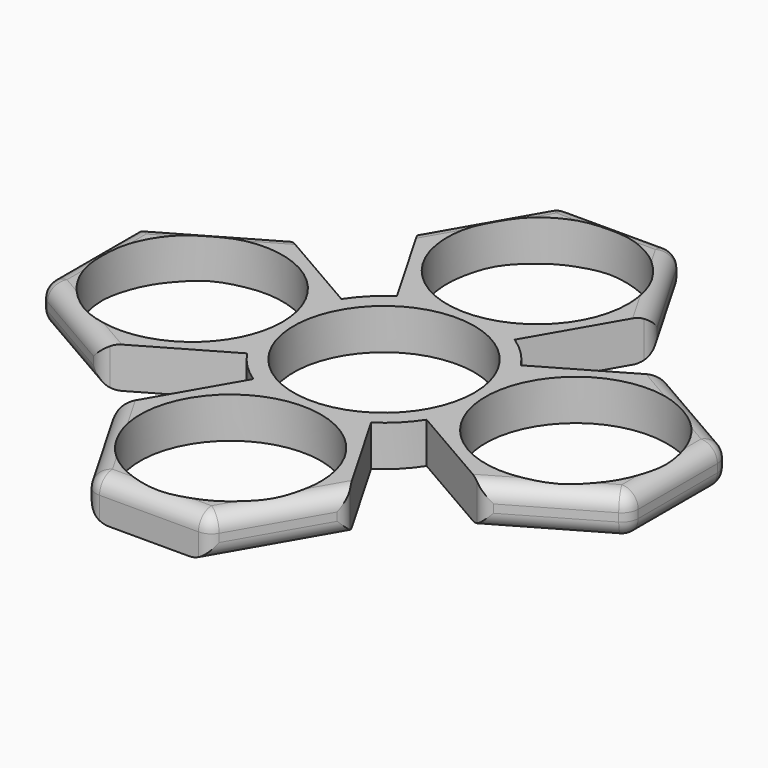
from build123d import *

# Parameters (mm, degrees)
F1_DEPTH      = 5
F2_R          = 11.075
F3_DEPTH      = 5
F4_T1_DEPTH   = 5.8867513459
F4_T3_DEPTH   = 10.7735026919
F4_T5_DEPTH   = 1
F4_T7_DEPTH   = 12.124355653
F4_T9_DEPTH   = 18.2790561914
F4_T11_DEPTH  = 18.2790561914
F4_T13_DEPTH  = 24.4337567297
F4_T15_DEPTH  = 12.124355653
F4_T17_DEPTH  = 24.4337567297
F4_T19_DEPTH  = 18.2790561914
F4_T21_DEPTH  = 18.2790561914
F4_T23_DEPTH  = 18.2790561914
F4_T25_DEPTH  = 24.4337567297
F4_T27_DEPTH  = 18.2790561914
F4_T29_DEPTH  = 18.2790561914
F4_T31_DEPTH  = 18.2790561914
F4_T36_DEPTH  = 2
F4_T42_DEPTH  = 2
F4_T48_DEPTH  = 2
F4_T54_DEPTH  = 2
F4_T60_DEPTH  = 2
F4_T66_DEPTH  = 2
F4_T72_DEPTH  = 2
F4_T78_DEPTH  = 2
F4_T84_DEPTH  = 2
F4_T90_DEPTH  = 2
F4_T96_DEPTH  = 2
F4_T102_DEPTH = 2


# Not quite as in the source:
# - a fillet or chamfer that OpenCascade refuses, or shapes differently, is made with other operations: its cross-section is extruded or revolved along the edge and cut away or added


with BuildPart() as f1:
    # F0 (on Top) → F1 (new body)
    with BuildSketch(Plane.XY):
        with BuildLine():
            ThreePointArc((-11, -7.2057268891), (-13.15, 0), (-11, 7.2057268891))
            Line((-11, 7.2057268891), (-11, 7.2168783649))
            Line((-11, 7.2168783649), (-23.5, 14.4337567297))
            Line((-23.5, 14.4337567297), (-36, 7.2168783649))
            Line((-36, 7.2168783649), (-36, -7.2168783649))
            Line((-36, -7.2168783649), (-23.5, -14.4337567297))
            Line((-23.5, -14.4337567297), (-11, -7.2168783649))
            Line((-11, -7.2168783649), (-11, -7.2057268891))
        make_face()
        with BuildLine():
            ThreePointArc((0, -11), (7.7781745931, -7.7781745931), (11, 0))
            ThreePointArc((11, 0), (7.7781745931, 7.7781745931), (0, 11))
            ThreePointArc((0, 11), (-7.7781745931, 7.7781745931), (-11, 0))
            ThreePointArc((-11, 0), (-7.7781745931, -7.7781745931), (0, -11))
        make_face()
        with BuildLine():
            Line((-11, -7.2057268891), (-11, 0))
            Line((-11, 0), (-11, 7.2057268891))
            ThreePointArc((-11, 7.2057268891), (-13.15, 0), (-11, -7.2057268891))
        make_face()
        with BuildLine():
            ThreePointArc((-7.2057268891, 11), (0, 13.15), (7.2057268891, 11))
            Line((7.2057268891, 11), (7.2168783649, 11))
            Line((7.2168783649, 11), (14.4337567297, 23.5))
            Line((14.4337567297, 23.5), (7.2168783649, 36))
            Line((7.2168783649, 36), (-7.2168783649, 36))
            Line((-7.2168783649, 36), (-14.4337567297, 23.5))
            Line((-14.4337567297, 23.5), (-7.2168783649, 11))
            Line((-7.2168783649, 11), (-7.2057268891, 11))
        make_face()
        with BuildLine():
            ThreePointArc((7.2057268891, -11), (0, -13.15), (-7.2057268891, -11))
            Line((-7.2057268891, -11), (-7.2168783649, -11))
            Line((-7.2168783649, -11), (-14.4337567297, -23.5))
            Line((-14.4337567297, -23.5), (-7.2168783649, -36))
            Line((-7.2168783649, -36), (7.2168783649, -36))
            Line((7.2168783649, -36), (14.4337567297, -23.5))
            Line((14.4337567297, -23.5), (7.2168783649, -11))
            Line((7.2168783649, -11), (7.2057268891, -11))
        make_face()
        with BuildLine():
            ThreePointArc((0, 11), (7.7781745931, 7.7781745931), (11, 0))
            Line((11, 0), (11, 7.2057268891))
            ThreePointArc((11, 7.2057268891), (9.2984541726, 9.2984541726), (7.2057268891, 11))
            Line((7.2057268891, 11), (0, 11))
        make_face()
        with BuildLine():
            ThreePointArc((13.15, 0), (12.6010416236, -3.7598204744), (11, -7.2057268891))
            Line((11, -7.2057268891), (11, -7.2168783649))
            Line((11, -7.2168783649), (23.5, -14.4337567297))
            Line((23.5, -14.4337567297), (36, -7.2168783649))
            Line((36, -7.2168783649), (36, 7.2168783649))
            Line((36, 7.2168783649), (23.5, 14.4337567297))
            Line((23.5, 14.4337567297), (11, 7.2168783649))
            Line((11, 7.2168783649), (11, 7.2057268891))
            ThreePointArc((11, 7.2057268891), (12.6010416236, 3.7598204744), (13.15, 0))
        make_face()
        with BuildLine():
            Line((11, 7.2057268891), (11, 0))
            Line((11, 0), (11, -7.2057268891))
            ThreePointArc((11, -7.2057268891), (12.6010416236, -3.7598204744), (13.15, 0))
            ThreePointArc((13.15, 0), (12.6010416236, 3.7598204744), (11, 7.2057268891))
        make_face()
        with BuildLine():
            Line((7.2057268891, -11), (0, -11))
            Line((0, -11), (-7.2057268891, -11))
            ThreePointArc((-7.2057268891, -11), (0, -13.15), (7.2057268891, -11))
        make_face()
        with BuildLine():
            Line((-7.2057268891, -11), (0, -11))
            ThreePointArc((0, -11), (-7.7781745931, -7.7781745931), (-11, 0))
            Line((-11, 0), (-11, -7.2057268891))
            ThreePointArc((-11, -7.2057268891), (-9.2984541726, -9.2984541726), (-7.2057268891, -11))
        make_face()
        with BuildLine():
            ThreePointArc((-11, 0), (-7.7781745931, 7.7781745931), (0, 11))
            Line((0, 11), (-7.2057268891, 11))
            ThreePointArc((-7.2057268891, 11), (-9.2984541726, 9.2984541726), (-11, 7.2057268891))
            Line((-11, 7.2057268891), (-11, 0))
        make_face()
        with BuildLine():
            Line((11, -7.2057268891), (11, 0))
            ThreePointArc((11, 0), (7.7781745931, -7.7781745931), (0, -11))
            Line((0, -11), (7.2057268891, -11))
            ThreePointArc((7.2057268891, -11), (9.2984541726, -9.2984541726), (11, -7.2057268891))
        make_face()
        with BuildLine():
            Line((-7.2057268891, 11), (0, 11))
            Line((0, 11), (7.2057268891, 11))
            ThreePointArc((7.2057268891, 11), (0, 13.15), (-7.2057268891, 11))
        make_face()
    extrude(amount=F1_DEPTH)

    # F2 (on face) → F3 (cut)
    with BuildSketch(Plane.XY.offset(5)):
        Circle(F2_R)
        with Locations((0, 23.5)):
            Circle(F2_R)
        with Locations((23.5, 0)):
            Circle(F2_R)
        with Locations((-23.5, 0)):
            Circle(F2_R)
        with Locations((0, -23.5)):
            Circle(F2_R)
    extrude(amount=-F3_DEPTH, mode=Mode.SUBTRACT)

    # F4: fillet of radius 2 on 38 edges, made by hand

    # F4_s2 → F4_t1 (cut)
    with BuildSketch(Plane.XY.offset(-2.8867513459)):
        with BuildLine():
            ThreePointArc((-7.7942286341, -35), (-7.0621778265, -35.7320508076), (-6.0621778265, -36))
            Line((-6.0621778265, -36), (-7.2168783649, -36))
            Line((-7.2168783649, -36), (-7.7942286341, -35))
        make_face()
        with BuildLine():
            ThreePointArc((6.0621778265, -36), (7.0621778265, -35.7320508076), (7.7942286341, -35))
            Line((7.7942286341, -35), (7.2168783649, -36))
            Line((7.2168783649, -36), (6.0621778265, -36))
        make_face()
    extrude(amount=F4_T1_DEPTH, mode=Mode.SUBTRACT)

    # F4_s4 → F4_t3 (cut)
    with BuildSketch(Plane.XY.offset(-2.8867513459)):
        with BuildLine():
            ThreePointArc((13.8564064606, -24.5), (14.124355653, -23.5), (13.8564064606, -22.5))
            Line((13.8564064606, -22.5), (14.4337567297, -23.5))
            Line((14.4337567297, -23.5), (13.8564064606, -24.5))
        make_face()
        with BuildLine():
            ThreePointArc((-13.8564064606, -22.5), (-14.124355653, -23.5), (-13.8564064606, -24.5))
            Line((-13.8564064606, -24.5), (-14.4337567297, -23.5))
            Line((-14.4337567297, -23.5), (-13.8564064606, -22.5))
        make_face()
        with BuildLine():
            ThreePointArc((-24.5, -13.8564064606), (-23.5, -14.124355653), (-22.5, -13.8564064606))
            Line((-22.5, -13.8564064606), (-23.5, -14.4337567297))
            Line((-23.5, -14.4337567297), (-24.5, -13.8564064606))
        make_face()
        with BuildLine():
            ThreePointArc((24.5, -13.8564064606), (23.5, -14.124355653), (22.5, -13.8564064606))
            Line((22.5, -13.8564064606), (23.5, -14.4337567297))
            Line((23.5, -14.4337567297), (24.5, -13.8564064606))
        make_face()
        with BuildLine():
            ThreePointArc((-13.8564064606, 22.5), (-14.124355653, 23.5), (-13.8564064606, 24.5))
            Line((-13.8564064606, 24.5), (-14.4337567297, 23.5))
            Line((-14.4337567297, 23.5), (-13.8564064606, 22.5))
        make_face()
        with BuildLine():
            ThreePointArc((13.8564064606, 24.5), (14.124355653, 23.5), (13.8564064606, 22.5))
            Line((13.8564064606, 22.5), (14.4337567297, 23.5))
            Line((14.4337567297, 23.5), (13.8564064606, 24.5))
        make_face()
        with BuildLine():
            ThreePointArc((-22.5, 13.8564064606), (-23.5, 14.124355653), (-24.5, 13.8564064606))
            Line((-24.5, 13.8564064606), (-23.5, 14.4337567297))
            Line((-23.5, 14.4337567297), (-22.5, 13.8564064606))
        make_face()
        with BuildLine():
            ThreePointArc((22.5, 13.8564064606), (23.5, 14.124355653), (24.5, 13.8564064606))
            Line((24.5, 13.8564064606), (23.5, 14.4337567297))
            Line((23.5, 14.4337567297), (22.5, 13.8564064606))
        make_face()
    extrude(amount=F4_T3_DEPTH, mode=Mode.SUBTRACT)

    # F4_s6 → F4_t5 (cut)
    with BuildSketch(Plane.XY.offset(2)):
        with BuildLine():
            ThreePointArc((-36, -6.0621778265), (-35.7320508076, -7.0621778265), (-35, -7.7942286341))
            Line((-35, -7.7942286341), (-36, -7.2168783649))
            Line((-36, -7.2168783649), (-36, -6.0621778265))
        make_face()
        with BuildLine():
            ThreePointArc((36, -6.0621778265), (35.7320508076, -7.0621778265), (35, -7.7942286341))
            Line((35, -7.7942286341), (36, -7.2168783649))
            Line((36, -7.2168783649), (36, -6.0621778265))
        make_face()
        with BuildLine():
            ThreePointArc((35, 7.7942286341), (35.7320508076, 7.0621778265), (36, 6.0621778265))
            Line((36, 6.0621778265), (36, 7.2168783649))
            Line((36, 7.2168783649), (35, 7.7942286341))
        make_face()
        with BuildLine():
            ThreePointArc((-7.7942286341, 35), (-7.0621778265, 35.7320508076), (-6.0621778265, 36))
            Line((-6.0621778265, 36), (-7.2168783649, 36))
            Line((-7.2168783649, 36), (-7.7942286341, 35))
        make_face()
        with BuildLine():
            ThreePointArc((6.0621778265, 36), (7.0621778265, 35.7320508076), (7.7942286341, 35))
            Line((7.7942286341, 35), (7.2168783649, 36))
            Line((7.2168783649, 36), (6.0621778265, 36))
        make_face()
    extrude(amount=F4_T5_DEPTH, mode=Mode.SUBTRACT)

    # F4_s8 → F4_t7 (cut)
    with BuildSketch(Plane.XZ.offset(-6.0621778265)):
        with BuildLine():
            ThreePointArc((34, 5), (35.4142135624, 4.4142135624), (36, 3))
            Line((36, 3), (36, 5))
            Line((36, 5), (34, 5))
        make_face()
        with BuildLine():
            ThreePointArc((34, 0), (35.4142135624, 0.5857864376), (36, 2))
            Line((36, 2), (36, 0))
            Line((36, 0), (34, 0))
        make_face()
    extrude(amount=F4_T7_DEPTH, mode=Mode.SUBTRACT)

    # F4_s10 → F4_t9 (cut)
    with BuildSketch(Plane(origin=(7.0448729811, 4.067359312, 0), x_dir=(0, 0, 1), z_dir=(0.8660254038, 0.5, 0))):
        with BuildLine():
            ThreePointArc((5, 22.25), (4.4142135624, 23.6642135624), (3, 24.25))
            Line((3, 24.25), (5, 24.25))
            Line((5, 24.25), (5, 22.25))
        make_face()
        with BuildLine():
            ThreePointArc((0, 22.25), (0.5857864376, 23.6642135624), (2, 24.25))
            Line((2, 24.25), (0, 24.25))
            Line((0, 24.25), (0, 22.25))
        make_face()
    extrude(amount=F4_T9_DEPTH, mode=Mode.SUBTRACT)

    # F4_s12 → F4_t11 (cut)
    with BuildSketch(Plane(origin=(-13.2068874077, -22.875, 0), x_dir=(0, 0, 1), z_dir=(0.5, 0.8660254038, 0))):
        with BuildLine():
            ThreePointArc((5, 22.25), (4.4142135624, 23.6642135624), (3, 24.25))
            Line((3, 24.25), (5, 24.25))
            Line((5, 24.25), (5, 22.25))
        make_face()
    extrude(amount=F4_T11_DEPTH, mode=Mode.SUBTRACT)

    # F4_s14 → F4_t13 (cut)
    with BuildSketch(Plane(origin=(-16.2842376769, -28.2051270189, 0), x_dir=(0, 0, 1), z_dir=(0.5, 0.8660254038, 0))):
        with BuildLine():
            ThreePointArc((0, 22.25), (0.5857864376, 23.6642135624), (2, 24.25))
            Line((2, 24.25), (0, 24.25))
            Line((0, 24.25), (0, 22.25))
        make_face()
    extrude(amount=F4_T13_DEPTH, mode=Mode.SUBTRACT)

    # F4_s16 → F4_t15 (cut)
    with BuildSketch(Plane.YZ.offset(-6.0621778265)):
        with BuildLine():
            ThreePointArc((-34, 5), (-35.4142135624, 4.4142135624), (-36, 3))
            Line((-36, 3), (-36, 5))
            Line((-36, 5), (-34, 5))
        make_face()
        with BuildLine():
            ThreePointArc((34, 0), (35.4142135624, 0.5857864376), (36, 2))
            Line((36, 2), (36, 0))
            Line((36, 0), (34, 0))
        make_face()
        with BuildLine():
            ThreePointArc((34, 5), (35.4142135624, 4.4142135624), (36, 3))
            Line((36, 3), (36, 5))
            Line((36, 5), (34, 5))
        make_face()
    extrude(amount=F4_T15_DEPTH, mode=Mode.SUBTRACT)

    # F4_s18 → F4_t17 (cut)
    with BuildSketch(Plane(origin=(4.067359312, -7.0448729811, 0), x_dir=(0, 0, 1), z_dir=(0.5, -0.8660254038, 0))):
        with BuildLine():
            ThreePointArc((0, 22.25), (0.5857864376, 23.6642135624), (2, 24.25))
            Line((2, 24.25), (0, 24.25))
            Line((0, 24.25), (0, 22.25))
        make_face()
    extrude(amount=F4_T17_DEPTH, mode=Mode.SUBTRACT)

    # F4_s20 → F4_t19 (cut)
    with BuildSketch(Plane(origin=(4.067359312, -7.0448729811, 0), x_dir=(0, 0, 1), z_dir=(0.5, -0.8660254038, 0))):
        with BuildLine():
            ThreePointArc((5, 22.25), (4.4142135624, 23.6642135624), (3, 24.25))
            Line((3, 24.25), (5, 24.25))
            Line((5, 24.25), (5, 22.25))
        make_face()
    extrude(amount=F4_T19_DEPTH, mode=Mode.SUBTRACT)

    # F4_s22 → F4_t21 (cut)
    with BuildSketch(Plane(origin=(-22.875, 13.2068874077, 0), x_dir=(0, 0, 1), z_dir=(0.8660254038, -0.5, 0))):
        with BuildLine():
            ThreePointArc((0, 22.25), (0.5857864376, 23.6642135624), (2, 24.25))
            Line((2, 24.25), (0, 24.25))
            Line((0, 24.25), (0, 22.25))
        make_face()
        with BuildLine():
            ThreePointArc((5, 22.25), (4.4142135624, 23.6642135624), (3, 24.25))
            Line((3, 24.25), (5, 24.25))
            Line((5, 24.25), (5, 22.25))
        make_face()
    extrude(amount=F4_T21_DEPTH, mode=Mode.SUBTRACT)

    # F4_s24 → F4_t23 (cut)
    with BuildSketch(Plane.XZ.offset(-12.2168783649)):
        with BuildLine():
            ThreePointArc((-34, 5), (-35.4142135624, 4.4142135624), (-36, 3))
            Line((-36, 3), (-36, 5))
            Line((-36, 5), (-34, 5))
        make_face()
        with BuildLine():
            ThreePointArc((-34, 0), (-35.4142135624, 0.5857864376), (-36, 2))
            Line((-36, 2), (-36, 0))
            Line((-36, 0), (-34, 0))
        make_face()
    extrude(amount=F4_T23_DEPTH, mode=Mode.SUBTRACT)

    # F4_s26 → F4_t25 (cut)
    with BuildSketch(Plane(origin=(-7.0448729811, -4.067359312, 0), x_dir=(0, 0, 1), z_dir=(-0.8660254038, -0.5, 0))):
        with BuildLine():
            ThreePointArc((2, 24.25), (0.5857864376, 23.6642135624), (0, 22.25))
            Line((0, 22.25), (0, 24.25))
            Line((0, 24.25), (2, 24.25))
        make_face()
        with BuildLine():
            ThreePointArc((3, 24.25), (4.4142135624, 23.6642135624), (5, 22.25))
            Line((5, 22.25), (5, 24.25))
            Line((5, 24.25), (3, 24.25))
        make_face()
    extrude(amount=F4_T25_DEPTH, mode=Mode.SUBTRACT)

    # F4_s28 → F4_t27 (cut)
    with BuildSketch(Plane(origin=(13.2068874077, 22.875, 0), x_dir=(0, 0, 1), z_dir=(-0.5, -0.8660254038, 0))):
        with BuildLine():
            ThreePointArc((0, 22.25), (0.5857864376, 23.6642135624), (2, 24.25))
            Line((2, 24.25), (0, 24.25))
            Line((0, 24.25), (0, 22.25))
        make_face()
        with BuildLine():
            ThreePointArc((5, 22.25), (4.4142135624, 23.6642135624), (3, 24.25))
            Line((3, 24.25), (5, 24.25))
            Line((5, 24.25), (5, 22.25))
        make_face()
    extrude(amount=F4_T27_DEPTH, mode=Mode.SUBTRACT)

    # F4_s30 → F4_t29 (cut)
    with BuildSketch(Plane(origin=(-4.067359312, 7.0448729811, 0), x_dir=(0, 0, 1), z_dir=(-0.5, 0.8660254038, 0))):
        with BuildLine():
            ThreePointArc((5, 22.25), (4.4142135624, 23.6642135624), (3, 24.25))
            Line((3, 24.25), (5, 24.25))
            Line((5, 24.25), (5, 22.25))
        make_face()
        with BuildLine():
            ThreePointArc((0, 22.25), (0.5857864376, 23.6642135624), (2, 24.25))
            Line((2, 24.25), (0, 24.25))
            Line((0, 24.25), (0, 22.25))
        make_face()
    extrude(amount=F4_T29_DEPTH, mode=Mode.SUBTRACT)

    # F4_s32 → F4_t31 (cut)
    with BuildSketch(Plane(origin=(22.875, -13.2068874077, 0), x_dir=(0, 0, 1), z_dir=(-0.8660254038, 0.5, 0))):
        with BuildLine():
            ThreePointArc((0, 22.25), (0.5857864376, 23.6642135624), (2, 24.25))
            Line((2, 24.25), (0, 24.25))
            Line((0, 24.25), (0, 22.25))
        make_face()
        with BuildLine():
            ThreePointArc((5, 22.25), (4.4142135624, 23.6642135624), (3, 24.25))
            Line((3, 24.25), (5, 24.25))
            Line((5, 24.25), (5, 22.25))
        make_face()
    extrude(amount=F4_T31_DEPTH, mode=Mode.SUBTRACT)


with BuildPart() as f4_tool34:
    # F4_s35 → F4_t36 (new body)
    with BuildSketch(Plane.XY.offset(3)):
        Polygon((-6.0621778265, -34), (-6.0621778265, -36), (-7.2168783649, -36), (-7.7942286341, -35), align=None)
    extrude(amount=F4_T36_DEPTH)

    # F4_s37 → F4_t38 (revolve, cut)
    with BuildSketch(Plane(origin=(-6.0621778265, -34, 3), x_dir=(0.5, 0.8660254038, 0), z_dir=(0.8660254038, -0.5, 0))):
        with BuildLine():
            ThreePointArc((0, -2), (2, 0), (0, 2))
            Line((0, 2), (0, -2))
        make_face()
    revolve(axis=Axis((-6.0621778265, -34, 3), (0, 0, 1)), mode=Mode.SUBTRACT)


with BuildPart() as f1_1:
    add(f1.part)

    # F4_t33: cut F4_tool34
    add(f4_tool34.part, mode=Mode.SUBTRACT)


with BuildPart() as f4_tool40:
    # F4_s41 → F4_t42 (new body)
    with BuildSketch(Plane.XY.offset(3)):
        Polygon((6.0621778265, -34), (6.0621778265, -36), (7.2168783649, -36), (7.7942286341, -35), align=None)
    extrude(amount=F4_T42_DEPTH)

    # F4_s43 → F4_t44 (revolve, cut)
    with BuildSketch(Plane(origin=(6.0621778265, -34, 3), x_dir=(-0.5, 0.8660254038, 0), z_dir=(0.8660254038, 0.5, 0))):
        with BuildLine():
            ThreePointArc((0, -2), (2, 0), (0, 2))
            Line((0, 2), (0, -2))
        make_face()
    revolve(axis=Axis((6.0621778265, -34, 3), (0, 0, 1)), mode=Mode.SUBTRACT)


with BuildPart() as f1_2:
    add(f1_1.part)

    # F4_t39: cut F4_tool40
    add(f4_tool40.part, mode=Mode.SUBTRACT)


with BuildPart() as f4_tool46:
    # F4_s47 → F4_t48 (new body)
    with BuildSketch(Plane.XY.offset(2)):
        Polygon((-34, -6.0621778265), (-36, -6.0621778265), (-36, -7.2168783649), (-35, -7.7942286341), align=None)
    extrude(amount=-F4_T48_DEPTH)

    # F4_s49 → F4_t50 (revolve, cut)
    with BuildSketch(Plane(origin=(-34, -6.0621778265, 2), x_dir=(0.8660254038, 0.5, 0), z_dir=(-0.5, 0.8660254038, 0))):
        with BuildLine():
            ThreePointArc((0, -2), (2, 0), (0, 2))
            Line((0, 2), (0, -2))
        make_face()
    revolve(axis=Axis((-34, -6.0621778265, 2), (0, 0, -1)), mode=Mode.SUBTRACT)


with BuildPart() as f1_3:
    add(f1_2.part)

    # F4_t45: cut F4_tool46
    add(f4_tool46.part, mode=Mode.SUBTRACT)


with BuildPart() as f4_tool52:
    # F4_s53 → F4_t54 (new body)
    with BuildSketch(Plane.XY.offset(3)):
        Polygon((-34, -6.0621778265), (-36, -6.0621778265), (-36, -7.2168783649), (-35, -7.7942286341), align=None)
    extrude(amount=F4_T54_DEPTH)

    # F4_s55 → F4_t56 (revolve, cut)
    with BuildSketch(Plane(origin=(-34, -6.0621778265, 3), x_dir=(0.8660254038, 0.5, 0), z_dir=(0.5, -0.8660254038, 0))):
        with BuildLine():
            ThreePointArc((0, -2), (2, 0), (0, 2))
            Line((0, 2), (0, -2))
        make_face()
    revolve(axis=Axis((-34, -6.0621778265, 3), (0, 0, 1)), mode=Mode.SUBTRACT)


with BuildPart() as f1_4:
    add(f1_3.part)

    # F4_t51: cut F4_tool52
    add(f4_tool52.part, mode=Mode.SUBTRACT)


with BuildPart() as f4_tool58:
    # F4_s59 → F4_t60 (new body)
    with BuildSketch(Plane.XY.offset(2)):
        Polygon((34, -6.0621778265), (36, -6.0621778265), (36, -7.2168783649), (35, -7.7942286341), align=None)
    extrude(amount=-F4_T60_DEPTH)

    # F4_s61 → F4_t62 (revolve, cut)
    with BuildSketch(Plane(origin=(34, -6.0621778265, 2), x_dir=(-0.8660254038, 0.5, 0), z_dir=(-0.5, -0.8660254038, 0))):
        with BuildLine():
            ThreePointArc((0, -2), (2, 0), (0, 2))
            Line((0, 2), (0, -2))
        make_face()
    revolve(axis=Axis((34, -6.0621778265, 2), (0, 0, -1)), mode=Mode.SUBTRACT)


with BuildPart() as f1_5:
    add(f1_4.part)

    # F4_t57: cut F4_tool58
    add(f4_tool58.part, mode=Mode.SUBTRACT)


with BuildPart() as f4_tool64:
    # F4_s65 → F4_t66 (new body)
    with BuildSketch(Plane.XY.offset(3)):
        Polygon((34, -6.0621778265), (36, -6.0621778265), (36, -7.2168783649), (35, -7.7942286341), align=None)
    extrude(amount=F4_T66_DEPTH)

    # F4_s67 → F4_t68 (revolve, cut)
    with BuildSketch(Plane(origin=(34, -6.0621778265, 3), x_dir=(-0.8660254038, 0.5, 0), z_dir=(0.5, 0.8660254038, 0))):
        with BuildLine():
            ThreePointArc((0, -2), (2, 0), (0, 2))
            Line((0, 2), (0, -2))
        make_face()
    revolve(axis=Axis((34, -6.0621778265, 3), (0, 0, 1)), mode=Mode.SUBTRACT)


with BuildPart() as f1_6:
    add(f1_5.part)

    # F4_t63: cut F4_tool64
    add(f4_tool64.part, mode=Mode.SUBTRACT)


with BuildPart() as f4_tool70:
    # F4_s71 → F4_t72 (new body)
    with BuildSketch(Plane.XY.offset(2)):
        Polygon((34, 6.0621778265), (35, 7.7942286341), (36, 7.2168783649), (36, 6.0621778265), align=None)
    extrude(amount=-F4_T72_DEPTH)

    # F4_s73 → F4_t74 (revolve, cut)
    with BuildSketch(Plane(origin=(34, 6.0621778265, 2), x_dir=(-0.8660254038, -0.5, 0), z_dir=(0.5, -0.8660254038, 0))):
        with BuildLine():
            ThreePointArc((0, -2), (2, 0), (0, 2))
            Line((0, 2), (0, -2))
        make_face()
    revolve(axis=Axis((34, 6.0621778265, 2), (0, 0, -1)), mode=Mode.SUBTRACT)


with BuildPart() as f1_7:
    add(f1_6.part)

    # F4_t69: cut F4_tool70
    add(f4_tool70.part, mode=Mode.SUBTRACT)


with BuildPart() as f4_tool76:
    # F4_s77 → F4_t78 (new body)
    with BuildSketch(Plane.XY.offset(3)):
        Polygon((34, 6.0621778265), (36, 6.0621778265), (36, 7.2168783649), (35, 7.7942286341), align=None)
    extrude(amount=F4_T78_DEPTH)

    # F4_s79 → F4_t80 (revolve, cut)
    with BuildSketch(Plane(origin=(34, 6.0621778265, 3), x_dir=(-0.8660254038, -0.5, 0), z_dir=(-0.5, 0.8660254038, 0))):
        with BuildLine():
            ThreePointArc((0, -2), (2, 0), (0, 2))
            Line((0, 2), (0, -2))
        make_face()
    revolve(axis=Axis((34, 6.0621778265, 3), (0, 0, 1)), mode=Mode.SUBTRACT)


with BuildPart() as f1_8:
    add(f1_7.part)

    # F4_t75: cut F4_tool76
    add(f4_tool76.part, mode=Mode.SUBTRACT)


with BuildPart() as f4_tool82:
    # F4_s83 → F4_t84 (new body)
    with BuildSketch(Plane.XY.offset(2)):
        Polygon((-6.0621778265, 34), (-6.0621778265, 36), (-7.2168783649, 36), (-7.7942286341, 35), align=None)
    extrude(amount=-F4_T84_DEPTH)

    # F4_s85 → F4_t86 (revolve, cut)
    with BuildSketch(Plane(origin=(-6.0621778265, 34, 2), x_dir=(0.5, -0.8660254038, 0), z_dir=(0.8660254038, 0.5, 0))):
        with BuildLine():
            ThreePointArc((0, -2), (2, 0), (0, 2))
            Line((0, 2), (0, -2))
        make_face()
    revolve(axis=Axis((-6.0621778265, 34, 2), (0, 0, -1)), mode=Mode.SUBTRACT)


with BuildPart() as f1_9:
    add(f1_8.part)

    # F4_t81: cut F4_tool82
    add(f4_tool82.part, mode=Mode.SUBTRACT)


with BuildPart() as f4_tool88:
    # F4_s89 → F4_t90 (new body)
    with BuildSketch(Plane.XY.offset(3)):
        Polygon((-6.0621778265, 34), (-6.0621778265, 36), (-7.2168783649, 36), (-7.7942286341, 35), align=None)
    extrude(amount=F4_T90_DEPTH)

    # F4_s91 → F4_t92 (revolve, cut)
    with BuildSketch(Plane(origin=(-6.0621778265, 34, 3), x_dir=(0.5, -0.8660254038, 0), z_dir=(-0.8660254038, -0.5, 0))):
        with BuildLine():
            ThreePointArc((0, -2), (2, 0), (0, 2))
            Line((0, 2), (0, -2))
        make_face()
    revolve(axis=Axis((-6.0621778265, 34, 3), (0, 0, 1)), mode=Mode.SUBTRACT)


with BuildPart() as f1_10:
    add(f1_9.part)

    # F4_t87: cut F4_tool88
    add(f4_tool88.part, mode=Mode.SUBTRACT)


with BuildPart() as f4_tool94:
    # F4_s95 → F4_t96 (new body)
    with BuildSketch(Plane.XY.offset(2)):
        Polygon((6.0621778265, 34), (6.0621778265, 36), (7.2168783649, 36), (7.7942286341, 35), align=None)
    extrude(amount=-F4_T96_DEPTH)

    # F4_s97 → F4_t98 (revolve, cut)
    with BuildSketch(Plane(origin=(6.0621778265, 34, 2), x_dir=(-0.5, -0.8660254038, 0), z_dir=(0.8660254038, -0.5, 0))):
        with BuildLine():
            ThreePointArc((0, -2), (2, 0), (0, 2))
            Line((0, 2), (0, -2))
        make_face()
    revolve(axis=Axis((6.0621778265, 34, 2), (0, 0, -1)), mode=Mode.SUBTRACT)


with BuildPart() as f1_11:
    add(f1_10.part)

    # F4_t93: cut F4_tool94
    add(f4_tool94.part, mode=Mode.SUBTRACT)


with BuildPart() as f4_tool100:
    # F4_s101 → F4_t102 (new body)
    with BuildSketch(Plane.XY.offset(3)):
        Polygon((6.0621778265, 34), (6.0621778265, 36), (7.2168783649, 36), (7.7942286341, 35), align=None)
    extrude(amount=F4_T102_DEPTH)

    # F4_s103 → F4_t104 (revolve, cut)
    with BuildSketch(Plane(origin=(6.0621778265, 34, 3), x_dir=(-0.5, -0.8660254038, 0), z_dir=(-0.8660254038, 0.5, 0))):
        with BuildLine():
            ThreePointArc((0, -2), (2, 0), (0, 2))
            Line((0, 2), (0, -2))
        make_face()
    revolve(axis=Axis((6.0621778265, 34, 3), (0, 0, 1)), mode=Mode.SUBTRACT)


with BuildPart() as f1_12:
    add(f1_11.part)

    # F4_t99: cut F4_tool100
    add(f4_tool100.part, mode=Mode.SUBTRACT)


solid = f1_12.part
